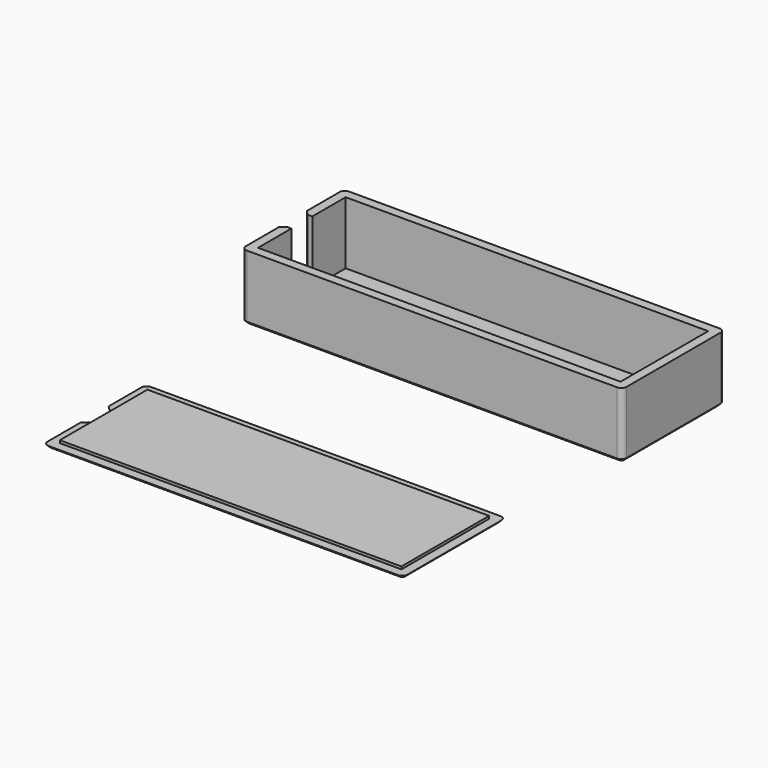
from build123d import *

# Parameters (mm, degrees)
F1_DEPTH  = 1
F2_DEPTH  = 25
F3_DEPTH  = 1
F4_DEPTH  = 2
F5_SIZE   = 0.99999
F5_2_SIZE = 0.99999


# Not quite as in the source:
# - a fillet or chamfer is up to 0.001 mm smaller than in the source, because OpenCascade refuses the exact size


with BuildPart() as f1:
    # F0 (on Top) → F1 (new body)
    with BuildSketch(Plane.XY):
        Polygon((-69.5, -5), (-69.5, -21), (69.5, -21), (69.5, 21), (-69.5, 21), (-69.5, 5), align=None)
    extrude(amount=F1_DEPTH)

    # F0 (on Top) → F2 (join)
    with BuildSketch(Plane.XY):
        with BuildLine():
            Line((69.5, -21), (-69.5, -21))
            Line((-69.5, -21), (-69.5, -5))
            Line((-69.5, -5), (-71.25, -5))
            Line((-71.25, -5), (-73, -6.75))
            Line((-73, -6.75), (-73, -22.5))
            ThreePointArc((-73, -22.5), (-72.4142135624, -23.9142135624), (-71, -24.5))
            Line((-71, -24.5), (71, -24.5))
            ThreePointArc((71, -24.5), (72.4142135624, -23.9142135624), (73, -22.5))
            Line((73, -22.5), (73, 22.5))
            ThreePointArc((73, 22.5), (72.4142135624, 23.9142135624), (71, 24.5))
            Line((71, 24.5), (-71, 24.5))
            ThreePointArc((-71, 24.5), (-72.4142135624, 23.9142135624), (-73, 22.5))
            Line((-73, 22.5), (-73, 6.75))
            Line((-73, 6.75), (-71.25, 5))
            Line((-71.25, 5), (-69.5, 5))
            Line((-69.5, 5), (-69.5, 21))
            Line((-69.5, 21), (69.5, 21))
            Line((69.5, 21), (69.5, -21))
        make_face()
    extrude(amount=F2_DEPTH)

    # F5 (size 1 in the source; OpenCascade refuses exactly that, so slightly less here)
    f5_edges = [f1.edges().sort_by_distance(p)[0] for p in [
        (-69.5, 0, 0),
        (-70.375, -5, 0),
        (-72.125, -5.875, 0),
        (-73, -14.625, 0),
        (-72.414214, -23.914214, 0),
        (0, -24.5, 0),
        (72.414214, -23.914214, 0),
        (73, 0, 0),
        (72.414214, 23.914214, 0),
        (0, 24.5, 0),
        (-72.414214, 23.914214, 0),
        (-73, 14.625, 0),
        (-72.125, 5.875, 0),
        (-70.375, 5, 0),
    ]]
    chamfer(f5_edges, length=F5_SIZE)


with BuildPart() as f3:
    # F0 (on Top) → F3 (new body)
    with BuildSketch(Plane.XY):
        with BuildLine():
            Line((65.5, -121), (-65.5, -121))
            Line((-65.5, -121), (-65.5, -105))
            Line((-65.5, -105), (-67.25, -105))
            Line((-67.25, -105), (-69, -106.75))
            Line((-69, -106.75), (-69, -122.5))
            ThreePointArc((-69, -122.5), (-68.4142135624, -123.9142135624), (-67, -124.5))
            Line((-67, -124.5), (67, -124.5))
            ThreePointArc((67, -124.5), (68.4142135624, -123.9142135624), (69, -122.5))
            Line((69, -122.5), (69, -77.5))
            ThreePointArc((69, -77.5), (68.4142135624, -76.0857864376), (67, -75.5))
            Line((67, -75.5), (-67, -75.5))
            ThreePointArc((-67, -75.5), (-68.4142135624, -76.0857864376), (-69, -77.5))
            Line((-69, -77.5), (-69, -93.25))
            Line((-69, -93.25), (-67.25, -95))
            Line((-67.25, -95), (-65.5, -95))
            Line((-65.5, -95), (-65.5, -79))
            Line((-65.5, -79), (65.5, -79))
            Line((65.5, -79), (65.5, -121))
        make_face()
    extrude(amount=F3_DEPTH)

    # F0 (on Top) → F4 (join)
    with BuildSketch(Plane.XY):
        Polygon((-65.5, -105), (-65.5, -121), (65.5, -121), (65.5, -79), (-65.5, -79), (-65.5, -95), align=None)
    extrude(amount=F4_DEPTH)

    # F5#2 (size 1 in the source; OpenCascade refuses exactly that, so slightly less here)
    f5_2_edges = [f3.edges().sort_by_distance(p)[0] for p in [
        (0, -124.5, 0),
        (-68.125, -105.875, 0),
        (-68.125, -94.125, 0),
        (-66.375, -95, 0),
        (-66.375, -105, 0),
        (-65.5, -100, 0),
    ]]
    chamfer(f5_2_edges, length=F5_2_SIZE)


solid = Compound([f1.part, f3.part])
